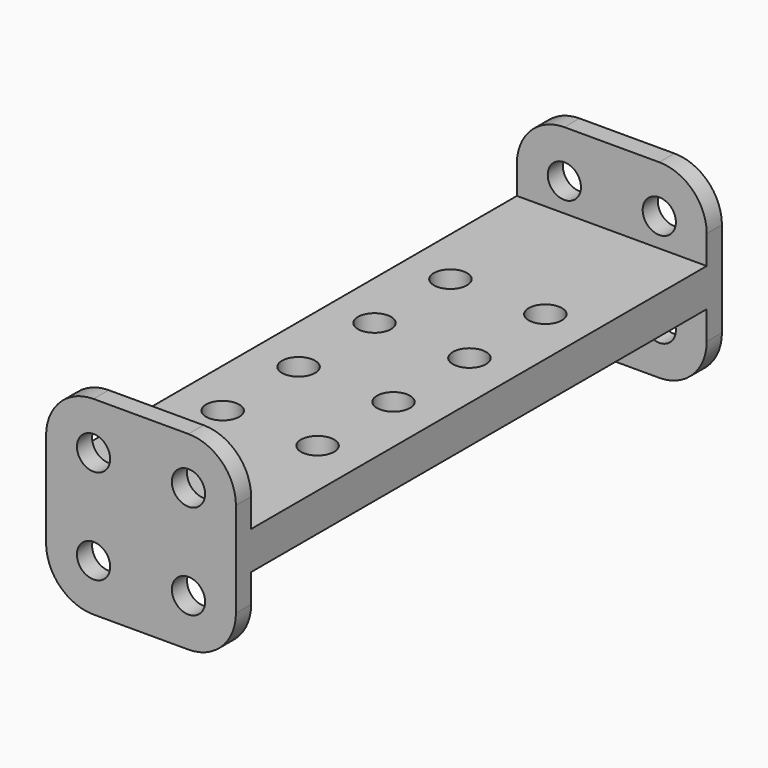
from build123d import *

# Parameters (mm, degrees)
F0_W     = 20
F0_H     = 60
F1_DEPTH = 2
F3_DEPTH = 2
F5_D     = 3.5
F6_W     = 20
F6_H     = 8
F6_H_2   = 4
F7_DEPTH = 2
F9_D     = 3.5
F10_R    = 5


# Not quite as in the source:
# - a feature names something its author has since deleted; it is built from what else it names


with BuildPart() as f1:
    # F0 (on Top) → F1 (new body, symmetric)
    with BuildSketch(Plane.XY):
        Rectangle(F0_W, F0_H)
    extrude(amount=F1_DEPTH, both=True)

    # F2 (on face) → F3 (join)
    with BuildSketch(Plane(origin=(0, 30, 0), x_dir=(-1, 0, 0), z_dir=(0, 1, 0))):
        Polygon((10, 2), (-2, 2), (2, -2), (10, -2), align=None)
        Polygon((-2, 2), (-10, 2), (-10, -2), (2, -2), align=None)
        Polygon((10, 10), (-10, 10), (-2, 2), (10, 2), align=None)
        Polygon((2, -2), (-10, -2), (-10, -10), (10, -10), align=None)
        Polygon((10, -2), (2, -2), (10, -10), align=None)
        Polygon((-2, 2), (-10, 10), (-10, 2), align=None)
    extrude(amount=F3_DEPTH)

    # F5 (through all)
    with Locations(Plane.XY.offset(2)):
        with Locations((5, 15), (-5, 15), (-5, 5), (5, 5), (5, -5), (-5, -5), (-5, -15), (5, -15)):
            Hole(F5_D / 2)

    # F6 (on face) → F7 (join)
    with BuildSketch(Plane.XZ.offset(30)):
        with Locations((0, 6)):
            Rectangle(F6_W, F6_H)
        Rectangle(F6_W, F6_H_2)
        with Locations((0, -6)):
            Rectangle(F6_W, F6_H)
    extrude(amount=F7_DEPTH)

    # F9 (through all)
    with Locations(Plane.XZ.offset(32)):
        with Locations((-5, 5), (5, 5), (5, -5), (-5, -5)):
            Hole(F9_D / 2)

    # F10
    f10_edges = [f1.edges().sort_by_distance(p)[0] for p in [
        (10, -31, 10),
        (10, -31, -10),
        (10, 31, 10),
        (10, 31, -10),
        (-10, 31, -10),
        (-10, 31, 10),
        (-10, -31, 10),
        (-10, -31, -10),
    ]]
    fillet(f10_edges, radius=F10_R)


solid = f1.part
